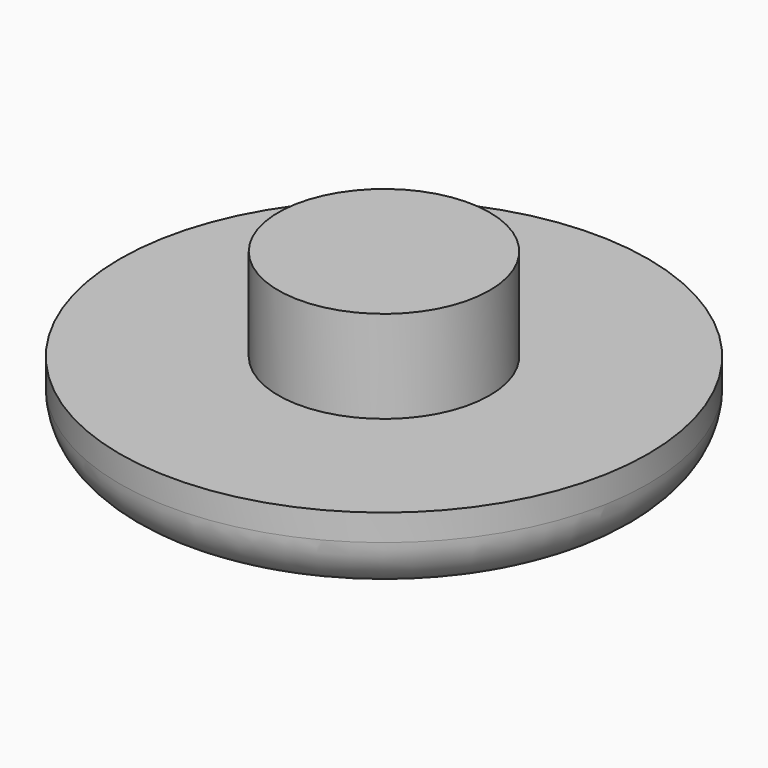
from build123d import *

# Parameters (mm, degrees)
F0_R         = 10
F1_DEPTH     = 3
F2_R         = 4
F3_DEPTH     = 3.5
F4_R         = 2
F5_TEXT_SIZE = 9.5993143347
F6_DEPTH     = 1.5


# Not quite as in the source:
# - Text() gives the source's letters only with a copy of the font that has no kerning and outlines rounded to 1/6400 em; it was checked with that copy


with BuildPart() as f1:
    # F0 (on Top) → F1 (new body)
    with BuildSketch(Plane.XY):
        Circle(F0_R)
    extrude(amount=F1_DEPTH)

    # F2 (on face) → F3 (join)
    with BuildSketch(Plane.XY.offset(3)):
        Circle(F2_R)
    extrude(amount=F3_DEPTH)

    # F4
    f4_edges = [f1.edges().sort_by_distance(p)[0] for p in [
        (-10, 0, 0),
    ]]
    fillet(f4_edges, radius=F4_R)

    # F5 (on face) → F6 (cut)
    with BuildSketch(Plane(origin=(0, 0, 0), x_dir=(1, 0, 0), z_dir=(0, 0, -1))):
        with Locations((-6.7488745187, -3.764608588)):
            Text('LM', F5_TEXT_SIZE, font='Arimo', font_style=FontStyle.ITALIC, text_align=(TextAlign.LEFT, TextAlign.BOTTOM))
    extrude(amount=-F6_DEPTH, mode=Mode.SUBTRACT)


solid = f1.part
